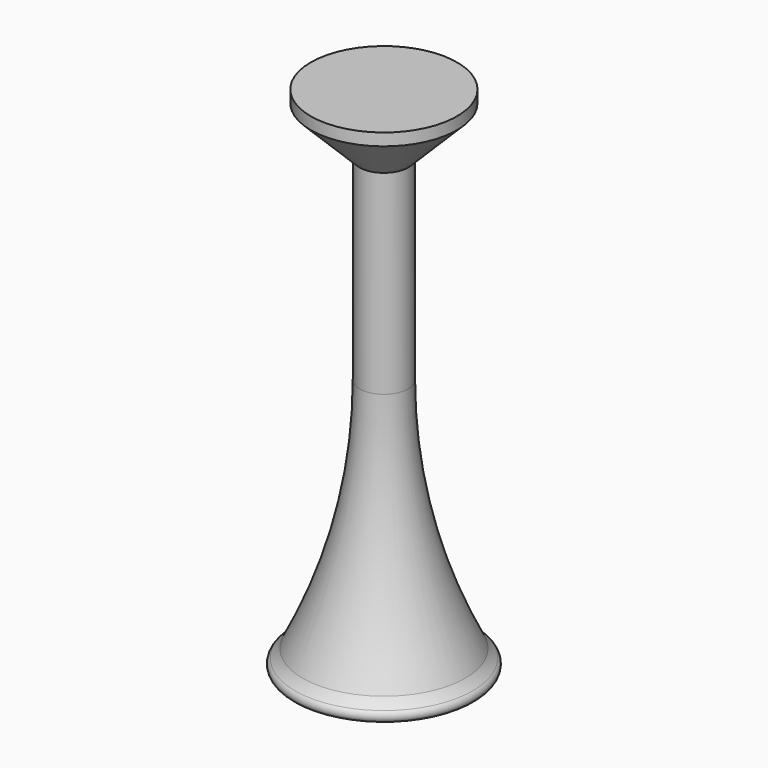
from build123d import *

# Parameters (mm, degrees)
F2_R    = 0.2
F3_SIZE = 0.39999


# Not quite as in the source:
# - a fillet or chamfer is up to 0.001 mm smaller than in the source, because OpenCascade refuses the exact size


with BuildPart() as f1:
    # F0 (on Front) → F1 (revolve)
    with BuildSketch(Plane.XZ):
        Polygon((-0.7, 0), (-0.65, 0), (0, 0.05), (0, 0.1), (-0.2, 0.1), (-0.7, 0.1), align=None)
        with BuildLine():
            ThreePointArc((-0.7, 0.1), (-0.75, 0.05), (-0.7, 0))
            Line((-0.7, 0), (-0.7, 0.1))
        make_face()
        with BuildLine():
            ThreePointArc((-0.2, 2.1), (-0.3268943744, 1.0692235936), (-0.7, 0.1))
            Line((-0.7, 0.1), (-0.2, 0.1))
            Line((-0.2, 0.1), (-0.2, 2.1))
        make_face()
        Polygon((-0.2, 0.1), (0, 0.1), (0, 4.1), (-0.2, 4.1), (-0.2, 2.1), align=None)
        Polygon((-0.2, 4.1), (0, 4.1), (0, 4.2), (-0.6, 4.2), (-0.6, 4.1), align=None)
    revolve(axis=Axis((0, 0, 2.1), (0, 0, 1)))

    # F2
    f2_edges = [f1.edges().sort_by_distance(p)[0] for p in [
        (0.7, 0, 0.1),
    ]]
    fillet(f2_edges, radius=F2_R)

    # F3 (size 0.4 in the source; OpenCascade refuses exactly that, so slightly less here)
    f3_edges = [f1.edges().sort_by_distance(p)[0] for p in [
        (0.2, 0, 4.1),
    ]]
    chamfer(f3_edges, length=F3_SIZE)


solid = f1.part
